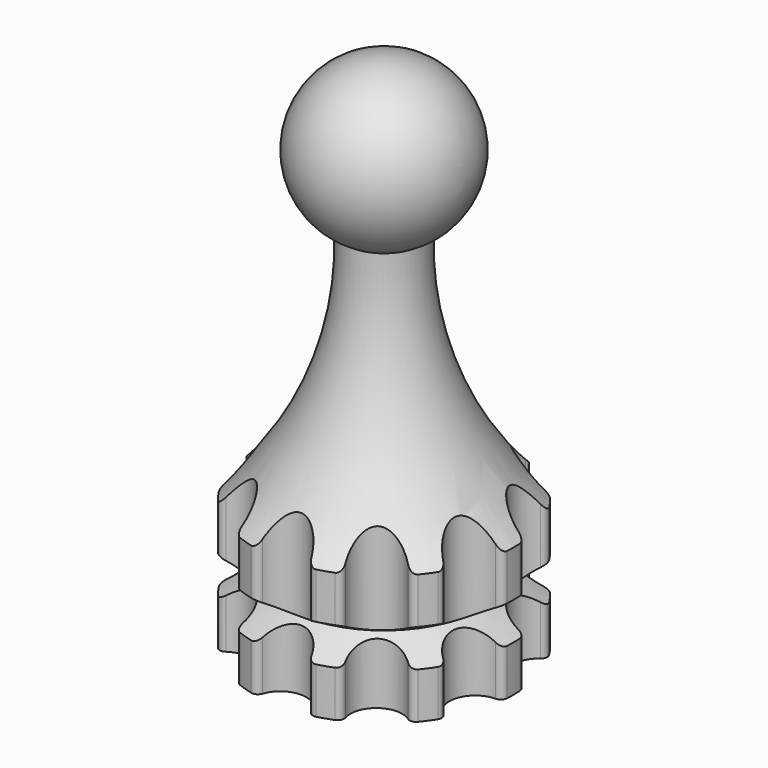
from build123d import *

# Parameters (mm, degrees)
F2_R        = 4
F3_DEPTH    = 25
F4_T1_DEPTH = 12.2770342332
F5_T1_DEPTH = 12.2770342332


# Not quite as in the source:
# - a fillet or chamfer that OpenCascade refuses, or shapes differently, is made with other operations: its cross-section is extruded or revolved along the edge and cut away or added


with BuildPart() as f1:
    # F0 (on Front) → F1 (revolve)
    with BuildSketch(Plane.XZ):
        with BuildLine():
            Line((0, 80), (0, 0))
            Line((0, 0), (20, 0))
            Line((20, 0), (20, 7.1132486541))
            Line((20, 7.1132486541), (15, 10))
            Line((15, 10), (20, 12.8867513459))
            Line((20, 12.8867513459), (20, 20))
            ThreePointArc((20, 20), (9.2781887481, 36.8408620554), (6, 56.5341439003))
            ThreePointArc((6, 56.5341439003), (12.1103922572, 70.5965140685), (0, 80))
        make_face()
    revolve(axis=Axis((0, 0, 40), (0, 0, -1)))

    # F2 (on face) → F3 (cut)
    with BuildSketch(Plane(origin=(0, 0, 0), x_dir=(1, 0, 0), z_dir=(0, 0, -1))):
        with Locations((0, 20)):
            Circle(F2_R)
        with Locations((-11.7557050458, 16.1803398875)):
            Circle(F2_R)
        with Locations((-19.0211303259, 6.1803398875)):
            Circle(F2_R)
        with Locations((-19.0211303259, -6.1803398875)):
            Circle(F2_R)
        with Locations((-11.7557050458, -16.1803398875)):
            Circle(F2_R)
        with Locations((0, -20)):
            Circle(F2_R)
        with Locations((11.7557050458, -16.1803398875)):
            Circle(F2_R)
        with Locations((19.0211303259, -6.1803398875)):
            Circle(F2_R)
        with Locations((19.0211303259, 6.1803398875)):
            Circle(F2_R)
        with Locations((11.7557050458, 16.1803398875)):
            Circle(F2_R)
    extrude(amount=-F3_DEPTH, mode=Mode.SUBTRACT)

    # F4: fillet of radius 1 on 20 edges, made by hand

    # F4_s2 → F4_t1 (cut)
    with BuildSketch(Plane.XY.offset(10.3048585564)):
        with BuildLine():
            ThreePointArc((-15.418561164, -12.7384446316), (-14.7790264009, -13.0928527193), (-14.0692474938, -12.9172858975))
            ThreePointArc((-14.0692474938, -12.9172858975), (-14.4217804008, -13.1983871378), (-14.7404379282, -13.5173773228))
            ThreePointArc((-14.7404379282, -13.5173773228), (-15.084528186, -13.1322888106), (-15.418561164, -12.7384446316))
        make_face()
        with BuildLine():
            ThreePointArc((-7.937432352, -17.3723103719), (-7.8850725774, -18.1016033582), (-7.3503833459, -18.60031894))
            ThreePointArc((-7.3503833459, -18.60031894), (-7.8281732856, -18.4043392441), (-8.3007439617, -18.1960888567))
            ThreePointArc((-8.3007439617, -18.1960888567), (-8.095836859, -17.7944541507), (-7.937432352, -17.3723103719))
        make_face()
        with BuildLine():
            ThreePointArc((-19.9613479021, -1.2428153251), (-19.6522692575, -1.9054465931), (-18.9748504708, -2.1806076246))
            ThreePointArc((-18.9748504708, -2.1806076246), (-19.4252827471, -2.2008096614), (-19.8705798284, -2.271575947))
            ThreePointArc((-19.8705798284, -2.271575947), (-19.9226053463, -1.7577816173), (-19.9613479021, -1.2428153251))
        make_face()
        with BuildLine():
            ThreePointArc((-16.6327054993, -9.3889886448), (-17.0190132138, -10.0097753679), (-16.8795782028, -10.7275271938))
            ThreePointArc((-16.8795782028, -10.7275271938), (-17.1509244088, -10.288138409), (-17.4108356104, -9.8418902325))
            ThreePointArc((-17.4108356104, -9.8418902325), (-17.008987325, -9.6374023029), (-16.6327054993, -9.3889886448))
        make_face()
        with BuildLine():
            ThreePointArc((-4.9864081189, -19.3684210526), (-4.2606977798, -19.2792341165), (-3.7896701703, -18.72))
            ThreePointArc((-3.7896701703, -18.72), (-3.9096481198, -19.1546293242), (-3.9799497484, -19.6))
            ThreePointArc((-3.9799497484, -19.6), (-4.4846739629, -19.4907080284), (-4.9864081189, -19.3684210526))
        make_face()
        with BuildLine():
            ThreePointArc((3.7896701703, -18.72), (4.2606977798, -19.2792341165), (4.9864081189, -19.3684210526))
            ThreePointArc((4.9864081189, -19.3684210526), (4.4846739629, -19.4907080284), (3.9799497484, -19.6))
            ThreePointArc((3.9799497484, -19.6), (3.9096481198, -19.1546293242), (3.7896701703, -18.72))
        make_face()
        with BuildLine():
            ThreePointArc((-16.8795782028, 10.7275271938), (-17.0190132138, 10.0097753679), (-16.6327054993, 9.3889886448))
            ThreePointArc((-16.6327054993, 9.3889886448), (-17.008987325, 9.6374023029), (-17.4108356104, 9.8418902325))
            ThreePointArc((-17.4108356104, 9.8418902325), (-17.1509244088, 10.288138409), (-16.8795782028, 10.7275271938))
        make_face()
        with BuildLine():
            ThreePointArc((-18.9748504708, 2.1806076246), (-19.6522692575, 1.9054465931), (-19.9613479021, 1.2428153251))
            ThreePointArc((-19.9613479021, 1.2428153251), (-19.9226053463, 1.7577816173), (-19.8705798284, 2.271575947))
            ThreePointArc((-19.8705798284, 2.271575947), (-19.4252827471, 2.2008096614), (-18.9748504708, 2.1806076246))
        make_face()
        with BuildLine():
            ThreePointArc((7.3503833459, -18.60031894), (7.8850725774, -18.1016033582), (7.937432352, -17.3723103719))
            ThreePointArc((7.937432352, -17.3723103719), (8.095836859, -17.7944541507), (8.3007439617, -18.1960888567))
            ThreePointArc((8.3007439617, -18.1960888567), (7.8281732856, -18.4043392441), (7.3503833459, -18.60031894))
        make_face()
        with BuildLine():
            ThreePointArc((14.0692474938, -12.9172858975), (14.7790264009, -13.0928527193), (15.418561164, -12.7384446316))
            ThreePointArc((15.418561164, -12.7384446316), (15.084528186, -13.1322888106), (14.7404379282, -13.5173773228))
            ThreePointArc((14.7404379282, -13.5173773228), (14.4217804008, -13.1983871378), (14.0692474938, -12.9172858975))
        make_face()
        with BuildLine():
            ThreePointArc((-7.3503833459, 18.60031894), (-7.8850725774, 18.1016033582), (-7.937432352, 17.3723103719))
            ThreePointArc((-7.937432352, 17.3723103719), (-8.095836859, 17.7944541507), (-8.3007439617, 18.1960888567))
            ThreePointArc((-8.3007439617, 18.1960888567), (-7.8281732856, 18.4043392441), (-7.3503833459, 18.60031894))
        make_face()
        with BuildLine():
            ThreePointArc((-14.0692474938, 12.9172858975), (-14.7790264009, 13.0928527193), (-15.418561164, 12.7384446316))
            ThreePointArc((-15.418561164, 12.7384446316), (-15.084528186, 13.1322888106), (-14.7404379282, 13.5173773228))
            ThreePointArc((-14.7404379282, 13.5173773228), (-14.4217804008, 13.1983871378), (-14.0692474938, 12.9172858975))
        make_face()
        with BuildLine():
            ThreePointArc((4.9864081189, 19.3684210526), (4.2606977798, 19.2792341165), (3.7896701703, 18.72))
            ThreePointArc((3.7896701703, 18.72), (3.9096481198, 19.1546293242), (3.9799497484, 19.6))
            ThreePointArc((3.9799497484, 19.6), (4.4846739629, 19.4907080284), (4.9864081189, 19.3684210526))
        make_face()
        with BuildLine():
            ThreePointArc((-3.7896701703, 18.72), (-4.2606977798, 19.2792341165), (-4.9864081189, 19.3684210526))
            ThreePointArc((-4.9864081189, 19.3684210526), (-4.4846739629, 19.4907080284), (-3.9799497484, 19.6))
            ThreePointArc((-3.9799497484, 19.6), (-3.9096481198, 19.1546293242), (-3.7896701703, 18.72))
        make_face()
        with BuildLine():
            ThreePointArc((15.418561164, 12.7384446316), (14.7790264009, 13.0928527193), (14.0692474938, 12.9172858975))
            ThreePointArc((14.0692474938, 12.9172858975), (14.4217804008, 13.1983871378), (14.7404379282, 13.5173773228))
            ThreePointArc((14.7404379282, 13.5173773228), (15.084528186, 13.1322888106), (15.418561164, 12.7384446316))
        make_face()
        with BuildLine():
            ThreePointArc((7.937432352, 17.3723103719), (7.8850725774, 18.1016033582), (7.3503833459, 18.60031894))
            ThreePointArc((7.3503833459, 18.60031894), (7.8281732856, 18.4043392441), (8.3007439617, 18.1960888567))
            ThreePointArc((8.3007439617, 18.1960888567), (8.095836859, 17.7944541507), (7.937432352, 17.3723103719))
        make_face()
        with BuildLine():
            ThreePointArc((16.6327054993, 9.3889886448), (17.0190132138, 10.0097753679), (16.8795782028, 10.7275271938))
            ThreePointArc((16.8795782028, 10.7275271938), (17.1509244088, 10.288138409), (17.4108356104, 9.8418902325))
            ThreePointArc((17.4108356104, 9.8418902325), (17.008987325, 9.6374023029), (16.6327054993, 9.3889886448))
        make_face()
        with BuildLine():
            ThreePointArc((18.9748504708, 2.1806076246), (19.6522692575, 1.9054465931), (19.9613479021, 1.2428153251))
            ThreePointArc((19.9613479021, 1.2428153251), (19.9226053463, 1.7577816173), (19.8705798284, 2.271575947))
            ThreePointArc((19.8705798284, 2.271575947), (19.4252827471, 2.2008096614), (18.9748504708, 2.1806076246))
        make_face()
        with BuildLine():
            ThreePointArc((16.8795782028, -10.7275271938), (17.0190132138, -10.0097753679), (16.6327054993, -9.3889886448))
            ThreePointArc((16.6327054993, -9.3889886448), (17.008987325, -9.6374023029), (17.4108356104, -9.8418902325))
            ThreePointArc((17.4108356104, -9.8418902325), (17.1509244088, -10.288138409), (16.8795782028, -10.7275271938))
        make_face()
        with BuildLine():
            ThreePointArc((18.9748504708, -2.1806076246), (19.6522692575, -1.9054465931), (19.9613479021, -1.2428153251))
            ThreePointArc((19.9613479021, -1.2428153251), (19.9226053463, -1.7577816173), (19.8705798284, -2.271575947))
            ThreePointArc((19.8705798284, -2.271575947), (19.4252827471, -2.2008096614), (18.9748504708, -2.1806076246))
        make_face()
    extrude(amount=F4_T1_DEPTH, mode=Mode.SUBTRACT)

    # F5: fillet of radius 1 on 20 edges, made by hand

    # F5_s2 → F5_t1 (cut)
    with BuildSketch(Plane.XY.offset(-2.5818927896)):
        with BuildLine():
            ThreePointArc((14.0692474938, 12.9172858975), (14.7790264009, 13.0928527193), (15.418561164, 12.7384446316))
            ThreePointArc((15.418561164, 12.7384446316), (15.084528186, 13.1322888106), (14.7404379282, 13.5173773228))
            ThreePointArc((14.7404379282, 13.5173773228), (14.4217804008, 13.1983871378), (14.0692474938, 12.9172858975))
        make_face()
        with BuildLine():
            ThreePointArc((7.3503833459, 18.60031894), (7.8850725774, 18.1016033582), (7.937432352, 17.3723103719))
            ThreePointArc((7.937432352, 17.3723103719), (8.095836859, 17.7944541507), (8.3007439617, 18.1960888567))
            ThreePointArc((8.3007439617, 18.1960888567), (7.8281732856, 18.4043392441), (7.3503833459, 18.60031894))
        make_face()
        with BuildLine():
            ThreePointArc((16.8795782028, 10.7275271938), (17.0190132138, 10.0097753679), (16.6327054993, 9.3889886448))
            ThreePointArc((16.6327054993, 9.3889886448), (17.008987325, 9.6374023029), (17.4108356104, 9.8418902325))
            ThreePointArc((17.4108356104, 9.8418902325), (17.1509244088, 10.288138409), (16.8795782028, 10.7275271938))
        make_face()
        with BuildLine():
            ThreePointArc((19.9613479021, 1.2428153251), (19.6522692575, 1.9054465931), (18.9748504708, 2.1806076246))
            ThreePointArc((18.9748504708, 2.1806076246), (19.4252827471, 2.2008096614), (19.8705798284, 2.271575947))
            ThreePointArc((19.8705798284, 2.271575947), (19.9226053463, 1.7577816173), (19.9613479021, 1.2428153251))
        make_face()
        with BuildLine():
            ThreePointArc((3.7896701703, 18.72), (4.2606977798, 19.2792341165), (4.9864081189, 19.3684210526))
            ThreePointArc((4.9864081189, 19.3684210526), (4.4846739629, 19.4907080284), (3.9799497484, 19.6))
            ThreePointArc((3.9799497484, 19.6), (3.9096481198, 19.1546293242), (3.7896701703, 18.72))
        make_face()
        with BuildLine():
            ThreePointArc((-4.9864081189, 19.3684210526), (-4.2606977798, 19.2792341165), (-3.7896701703, 18.72))
            ThreePointArc((-3.7896701703, 18.72), (-3.9096481198, 19.1546293242), (-3.9799497484, 19.6))
            ThreePointArc((-3.9799497484, 19.6), (-4.4846739629, 19.4907080284), (-4.9864081189, 19.3684210526))
        make_face()
        with BuildLine():
            ThreePointArc((-7.937432352, 17.3723103719), (-7.8850725774, 18.1016033582), (-7.3503833459, 18.60031894))
            ThreePointArc((-7.3503833459, 18.60031894), (-7.8281732856, 18.4043392441), (-8.3007439617, 18.1960888567))
            ThreePointArc((-8.3007439617, 18.1960888567), (-8.095836859, 17.7944541507), (-7.937432352, 17.3723103719))
        make_face()
        with BuildLine():
            ThreePointArc((-15.418561164, 12.7384446316), (-14.7790264009, 13.0928527193), (-14.0692474938, 12.9172858975))
            ThreePointArc((-14.0692474938, 12.9172858975), (-14.4217804008, 13.1983871378), (-14.7404379282, 13.5173773228))
            ThreePointArc((-14.7404379282, 13.5173773228), (-15.084528186, 13.1322888106), (-15.418561164, 12.7384446316))
        make_face()
        with BuildLine():
            ThreePointArc((-16.6327054993, 9.3889886448), (-17.0190132138, 10.0097753679), (-16.8795782028, 10.7275271938))
            ThreePointArc((-16.8795782028, 10.7275271938), (-17.1509244088, 10.288138409), (-17.4108356104, 9.8418902325))
            ThreePointArc((-17.4108356104, 9.8418902325), (-17.008987325, 9.6374023029), (-16.6327054993, 9.3889886448))
        make_face()
        with BuildLine():
            ThreePointArc((-19.9613479021, 1.2428153251), (-19.6522692575, 1.9054465931), (-18.9748504708, 2.1806076246))
            ThreePointArc((-18.9748504708, 2.1806076246), (-19.4252827471, 2.2008096614), (-19.8705798284, 2.271575947))
            ThreePointArc((-19.8705798284, 2.271575947), (-19.9226053463, 1.7577816173), (-19.9613479021, 1.2428153251))
        make_face()
        with BuildLine():
            ThreePointArc((16.6327054993, -9.3889886448), (17.0190132138, -10.0097753679), (16.8795782028, -10.7275271938))
            ThreePointArc((16.8795782028, -10.7275271938), (17.1509244088, -10.288138409), (17.4108356104, -9.8418902325))
            ThreePointArc((17.4108356104, -9.8418902325), (17.008987325, -9.6374023029), (16.6327054993, -9.3889886448))
        make_face()
        with BuildLine():
            ThreePointArc((19.9613479021, -1.2428153251), (19.6522692575, -1.9054465931), (18.9748504708, -2.1806076246))
            ThreePointArc((18.9748504708, -2.1806076246), (19.4252827471, -2.2008096614), (19.8705798284, -2.271575947))
            ThreePointArc((19.8705798284, -2.271575947), (19.9226053463, -1.7577816173), (19.9613479021, -1.2428153251))
        make_face()
        with BuildLine():
            ThreePointArc((7.937432352, -17.3723103719), (7.8850725774, -18.1016033582), (7.3503833459, -18.60031894))
            ThreePointArc((7.3503833459, -18.60031894), (7.8281732856, -18.4043392441), (8.3007439617, -18.1960888567))
            ThreePointArc((8.3007439617, -18.1960888567), (8.095836859, -17.7944541507), (7.937432352, -17.3723103719))
        make_face()
        with BuildLine():
            ThreePointArc((15.418561164, -12.7384446316), (14.7790264009, -13.0928527193), (14.0692474938, -12.9172858975))
            ThreePointArc((14.0692474938, -12.9172858975), (14.4217804008, -13.1983871378), (14.7404379282, -13.5173773228))
            ThreePointArc((14.7404379282, -13.5173773228), (15.084528186, -13.1322888106), (15.418561164, -12.7384446316))
        make_face()
        with BuildLine():
            ThreePointArc((-3.7896701703, -18.72), (-4.2606977798, -19.2792341165), (-4.9864081189, -19.3684210526))
            ThreePointArc((-4.9864081189, -19.3684210526), (-4.4846739629, -19.4907080284), (-3.9799497484, -19.6))
            ThreePointArc((-3.9799497484, -19.6), (-3.9096481198, -19.1546293242), (-3.7896701703, -18.72))
        make_face()
        with BuildLine():
            ThreePointArc((4.9864081189, -19.3684210526), (4.2606977798, -19.2792341165), (3.7896701703, -18.72))
            ThreePointArc((3.7896701703, -18.72), (3.9096481198, -19.1546293242), (3.9799497484, -19.6))
            ThreePointArc((3.9799497484, -19.6), (4.4846739629, -19.4907080284), (4.9864081189, -19.3684210526))
        make_face()
        with BuildLine():
            ThreePointArc((-14.0692474938, -12.9172858975), (-14.7790264009, -13.0928527193), (-15.418561164, -12.7384446316))
            ThreePointArc((-15.418561164, -12.7384446316), (-15.084528186, -13.1322888106), (-14.7404379282, -13.5173773228))
            ThreePointArc((-14.7404379282, -13.5173773228), (-14.4217804008, -13.1983871378), (-14.0692474938, -12.9172858975))
        make_face()
        with BuildLine():
            ThreePointArc((-7.3503833459, -18.60031894), (-7.8850725774, -18.1016033582), (-7.937432352, -17.3723103719))
            ThreePointArc((-7.937432352, -17.3723103719), (-8.095836859, -17.7944541507), (-8.3007439617, -18.1960888567))
            ThreePointArc((-8.3007439617, -18.1960888567), (-7.8281732856, -18.4043392441), (-7.3503833459, -18.60031894))
        make_face()
        with BuildLine():
            ThreePointArc((-18.9748504708, -2.1806076246), (-19.6522692575, -1.9054465931), (-19.9613479021, -1.2428153251))
            ThreePointArc((-19.9613479021, -1.2428153251), (-19.9226053463, -1.7577816173), (-19.8705798284, -2.271575947))
            ThreePointArc((-19.8705798284, -2.271575947), (-19.4252827471, -2.2008096614), (-18.9748504708, -2.1806076246))
        make_face()
        with BuildLine():
            ThreePointArc((-16.8795782028, -10.7275271938), (-17.0190132138, -10.0097753679), (-16.6327054993, -9.3889886448))
            ThreePointArc((-16.6327054993, -9.3889886448), (-17.008987325, -9.6374023029), (-17.4108356104, -9.8418902325))
            ThreePointArc((-17.4108356104, -9.8418902325), (-17.1509244088, -10.288138409), (-16.8795782028, -10.7275271938))
        make_face()
    extrude(amount=F5_T1_DEPTH, mode=Mode.SUBTRACT)


solid = f1.part
